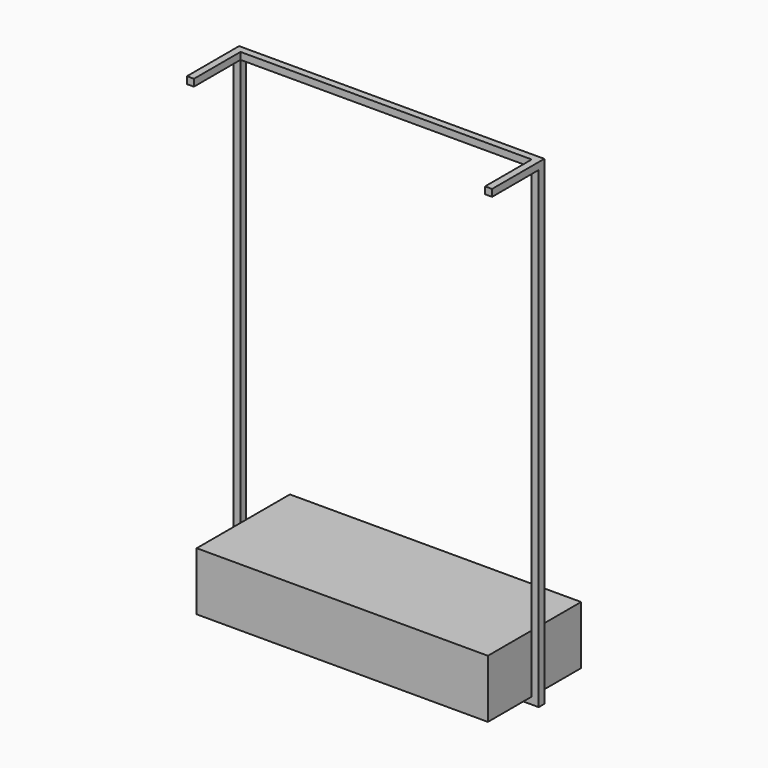
from build123d import *

# Parameters (mm, degrees)
F0_W     = 1250
F0_H     = 500
F1_DEPTH = 250
F2_W     = 1310
F2_H     = 2060
F2_W_2   = 1250
F2_H_2   = 2000
F3_DEPTH = 15
F4_W     = 1050
F4_H     = 300
F4_W_2   = 990
F4_H_2   = 240
F5_DEPTH = 30
F6_W     = 30
F6_H     = 30
F7_DEPTH = 250


# Not quite as in the source:
# - a feature of the source that left no trace in its solid (it failed there, or was rolled back) is left out


with BuildPart() as f1:
    # F0 (on Top) → F1 (new body)
    with BuildSketch(Plane.XY):
        Rectangle(F0_W, F0_H)
    extrude(amount=F1_DEPTH)


with BuildPart() as f3:
    # F2 (on Front) → F3 (new body, symmetric)
    with BuildSketch(Plane.XZ):
        with Locations((0, 1000)):
            Rectangle(F2_W, F2_H)
        with Locations((0, 1000)):
            Rectangle(F2_W_2, F2_H_2, mode=Mode.SUBTRACT)
    extrude(amount=F3_DEPTH, both=True)

    # F4 (on face) → F5 (join)
    with BuildSketch(Plane(origin=(0, 0, 0), x_dir=(1, 0, 0), z_dir=(0, 0, -1))):
        Rectangle(F4_W, F4_H)
        Rectangle(F4_W_2, F4_H_2, mode=Mode.SUBTRACT)
    extrude(amount=F5_DEPTH)

    # F6 (on face) → F7 (join)
    with BuildSketch(Plane.XZ.offset(15)):
        with Locations((640, 2015)):
            Rectangle(F6_W, F6_H)
        with Locations((-640, 2015)):
            Rectangle(F6_W, F6_H)
    extrude(amount=F7_DEPTH)


solid = Compound([f1.part, f3.part])
